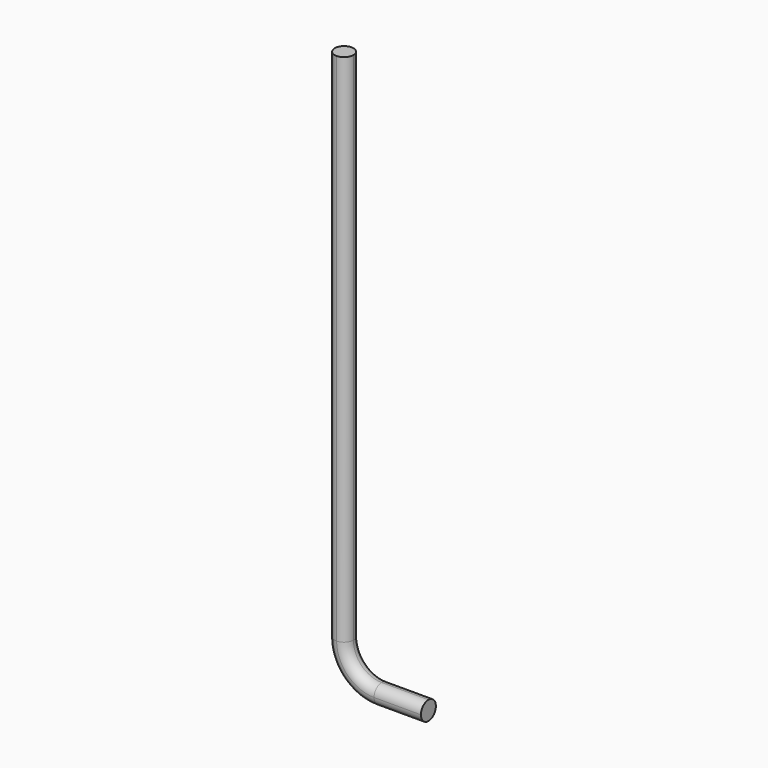
from build123d import *

# Parameters (mm, degrees)
F1_DEPTH = 20
F2_R     = 9.99999


# Not quite as in the source:
# - a fillet or chamfer is up to 0.001 mm smaller than in the source, because OpenCascade refuses the exact size


with BuildPart() as f1:
    # F0 (on Front) → F1 (new body)
    with BuildSketch(Plane.XZ):
        with BuildLine():
            Line((0, 600), (0, 50))
            ThreePointArc((0, 50), (14.6446609407, 14.6446609407), (50, 0))
            Line((50, 0), (100, 0))
            Line((100, 0), (100, 20))
            Line((100, 20), (50, 20))
            ThreePointArc((50, 20), (28.7867965644, 28.7867965644), (20, 50))
            Line((20, 50), (20, 600))
            Line((20, 600), (0, 600))
        make_face()
    extrude(amount=F1_DEPTH)

    # F2 (radius 10 in the source; OpenCascade refuses exactly that, so slightly less here)
    f2_edges = [f1.edges().sort_by_distance(p)[0] for p in [
        (0, -20, 325),
        (20, -20, 325),
        (20, 0, 325),
        (0, 0, 325),
    ]]
    fillet(f2_edges, radius=F2_R)


solid = f1.part
